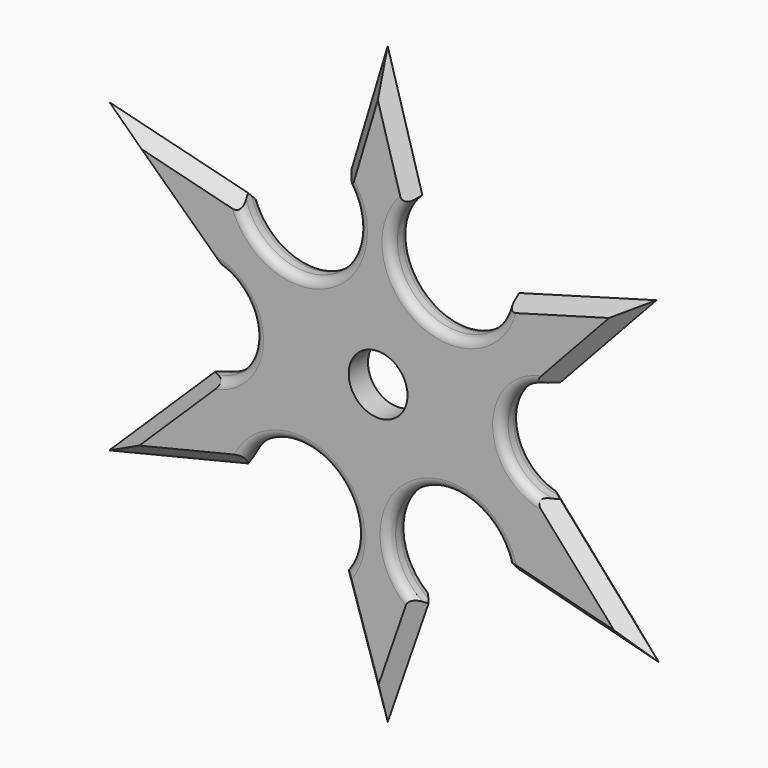
from build123d import *

# Parameters (mm, degrees)
F0_R         = 4.0240897433
F0_R_2       = 2.1702911965
F1_DEPTH     = 0.889
F2_DEPTH     = 0.889
F3_SIZE      = 1.016
F4_R         = 0.635
F5_T1_DEPTH  = 15.9932905978
F5_T3_DEPTH  = 16.1545129753
F5_T5_DEPTH  = 16.1936477888
F5_T7_DEPTH  = 16.3204160833
F5_T9_DEPTH  = 16.5038775979
F5_T11_DEPTH = 16.1754599615
F5_T13_DEPTH = 14.8813266149
F5_T15_DEPTH = 14.7778979971
F5_T17_DEPTH = 16.2458412717
F5_T19_DEPTH = 16.498961557
F5_T21_DEPTH = 14.852247235
F5_T23_DEPTH = 14.8224282878
F6_R         = 0.635


# Not quite as in the source:
# - a fillet or chamfer that OpenCascade refuses, or shapes differently, is made with other operations: its cross-section is extruded or revolved along the edge and cut away or added


with BuildPart() as f1:
    # F0 (on Front) → F1 (new body, symmetric)
    with BuildSketch(Plane.XZ):
        with BuildLine():
            ThreePointArc((-12.921775703, 3.9272087544), (-9.095056291, 0.1291059315), (-12.921775703, -3.6689968914))
            Line((-12.921775703, -3.6689968914), (-11.6317034987, -6.3241203273))
            Line((-11.6317034987, -6.3241203273), (-10.3416312944, -8.9792437632))
            ThreePointArc((-10.3416312944, -8.9792437632), (-3.7268534074, -6.4636823832), (-2.9634656604, -13.4993468649))
            Line((-2.9634656604, -13.4993468649), (0, -13.5794270365))
            Line((0, -13.5794270365), (3.1296215133, -13.6639971501))
            ThreePointArc((3.1296215133, -13.6639971501), (2.8041191173, -5.9768088987), (9.7185348855, -9.3516673562))
            Line((9.7185348855, -9.3516673562), (11.3201552942, -6.5125130277))
            Line((11.3201552942, -6.5125130277), (12.921775703, -3.6733586992))
            ThreePointArc((12.921775703, -3.6733586992), (9.0928589552, 0.1269250276), (12.921775703, 3.9272087544))
            Line((12.921775703, 3.9272087544), (11.3201552942, 6.4055448308))
            Line((11.3201552942, 6.4055448308), (9.7185348855, 8.8838809072))
            ThreePointArc((9.7185348855, 8.8838809072), (3.1603710023, 5.5177443003), (2.6637583381, 12.8725906642))
            Line((2.6637583381, 12.8725906642), (0, 12.8725906642))
            Line((0, 12.8725906642), (-2.7692650138, 12.8725906642))
            ThreePointArc((-2.7692650138, 12.8725906642), (-3.8215008101, 5.6879732844), (-10.3416312944, 8.8838809072))
            Line((-10.3416312944, 8.8838809072), (-11.6317034987, 6.4055448308))
            Line((-11.6317034987, 6.4055448308), (-12.921775703, 3.9272087544))
        make_face()
        Circle(F0_R, mode=Mode.SUBTRACT)
        Circle(F0_R)
        Circle(F0_R_2, mode=Mode.SUBTRACT)
    extrude(amount=F1_DEPTH, both=True)

    # F0 (on Front) → F2 (join, symmetric)
    with BuildSketch(Plane.XZ):
        Polygon((-16.3057108253, 8.9796162218), (-11.6317034987, 6.4055448308), (-10.3416312944, 8.8838809072), align=None)
        Polygon((-16.3057108253, 8.9796162218), (-12.921775703, 3.9272087544), (-11.6317034987, 6.4055448308), align=None)
        Polygon((-20.9797181518, 11.5536876128), (-12.921775703, 3.9272087544), (-16.3057108253, 8.9796162218), align=None)
        Polygon((-10.3416312944, 8.8838809072), (-20.9797181518, 11.5536876128), (-16.3057108253, 8.9796162218), align=None)
        Polygon((0, 17.4824267871), (-2.7692650138, 12.8725906642), (0, 12.8725906642), align=None)
        Polygon((0, 17.4824267871), (0, 12.8725906642), (2.6637583381, 12.8725906642), align=None)
        Polygon((2.6637583381, 12.8725906642), (0, 22.0922629099), (0, 17.4824267871), align=None)
        Polygon((0, 22.0922629099), (-2.7692650138, 12.8725906642), (0, 17.4824267871), align=None)
        Polygon((-16.378282755, -8.9792437632), (-20.9840265761, -11.5555872095), (-10.3416312944, -8.9792437632), align=None)
        Polygon((-16.378282755, -8.9792437632), (-12.921775703, -3.6689968914), (-20.9840265761, -11.5555872095), align=None)
        Polygon((-11.6317034987, -6.3241203273), (-12.921775703, -3.6689968914), (-16.378282755, -8.9792437632), align=None)
        Polygon((-10.3416312944, -8.9792437632), (-11.6317034987, -6.3241203273), (-16.378282755, -8.9792437632), align=None)
        Polygon((0, -18.7971512683), (-2.9634656604, -13.4993468649), (0, -22.6890025881), align=None)
        Polygon((0, -18.7971512683), (0, -22.6890025881), (3.1296215133, -13.6639971501), align=None)
        Polygon((3.1296215133, -13.6639971501), (0, -13.5794270365), (0, -18.7971512683), align=None)
        Polygon((0, -13.5794270365), (-2.9634656604, -13.4993468649), (0, -18.7971512683), align=None)
        Polygon((16.1898454279, -9.5265381722), (20.3846063865, -12.1228255452), (12.921775703, -3.6733586992), align=None)
        Polygon((12.921775703, -3.6733586992), (11.3201552942, -6.5125130277), (16.1898454279, -9.5265381722), align=None)
        Polygon((11.3201552942, -6.5125130277), (9.7185348855, -9.3516673562), (16.1898454279, -9.5265381722), align=None)
        Polygon((16.1898454279, -9.5265381722), (9.7185348855, -9.3516673562), (20.3846063865, -12.1228255452), align=None)
        Polygon((12.921775703, 3.9272087544), (20.2454214595, 11.8206291252), (15.7827883769, 9.113086978), align=None)
        Polygon((20.2454214595, 11.8206291252), (9.7185348855, 8.8838809072), (15.7827883769, 9.113086978), align=None)
        Polygon((15.7827883769, 9.113086978), (9.7185348855, 8.8838809072), (11.3201552942, 6.4055448308), align=None)
        Polygon((15.7827883769, 9.113086978), (11.3201552942, 6.4055448308), (12.921775703, 3.9272087544), align=None)
    extrude(amount=F2_DEPTH, both=True)

    # F3
    f3_edges = [f1.edges().sort_by_distance(p)[0] for p in [
        (-15.660675, -0.889, 10.218784),
        (-16.950747, -0.889, 7.740448),
        (-1.384633, -0.889, 17.482427),
        (1.331879, -0.889, 17.482427),
        (14.981978, -0.889, 10.352255),
        (16.583599, -0.889, 7.873919),
        (16.653191, -0.889, -7.898092),
        (15.051571, -0.889, -10.737246),
        (1.564811, -0.889, -18.1765),
        (-1.481733, -0.889, -18.094175),
        (-15.662829, -0.889, -10.267415),
        (-16.952901, -0.889, -7.612292),
    ]]
    chamfer(f3_edges, length=F3_SIZE)

    # F4
    f4_edges = [f1.edges().sort_by_distance(p)[0] for p in [
        (-3.69199, -0.889, -6.485261),
        (2.770724, -0.889, -5.998879),
        (9.093189, -0.889, 0.07683),
        (3.156805, -0.889, 5.519763),
        (-3.847037, -0.889, 5.674627),
        (-9.0961, -0.889, 0.040071),
    ]]
    fillet(f4_edges, radius=F4_R)

    # F5: chamfer of 1.016 on 12 edges, made by hand

    # F5_s2 → F5_t1 (cut)
    with BuildSketch(Plane(origin=(6.1587132778, 0, 6.6378569447), x_dir=(0, 1, 0), z_dir=(0.6801538719, 0, 0.7330693764))):
        Polygon((0.889, -5.7854518163), (-0.127, -6.8014518163), (0.889, -6.8014518163), align=None)
    extrude(amount=F5_T1_DEPTH, mode=Mode.SUBTRACT)

    # F5_s4 → F5_t3 (cut)
    with BuildSketch(Plane(origin=(24.3598265124, 0, 6.7958058252), x_dir=(0, 1, 0), z_dir=(-0.9632196934, 0, -0.2687151323))):
        Polygon((0.889, -4.9296116562), (-0.127, -5.9456116562), (0.889, -5.9456116562), align=None)
    extrude(amount=F5_T3_DEPTH, mode=Mode.SUBTRACT)

    # F5_s6 → F5_t5 (cut)
    with BuildSketch(Plane(origin=(-9.2920779296, 0, 2.3320031409), x_dir=(0, 1, 0), z_dir=(-0.9699214568, 0, 0.2434180924))):
        Polygon((-0.127, -6.0993265498), (0.889, -5.0833265498), (0.889, -6.0993265498), align=None)
    extrude(amount=F5_T5_DEPTH, mode=Mode.SUBTRACT)

    # F5_s8 → F5_t7 (cut)
    with BuildSketch(Plane(origin=(-18.7323182554, 0, 17.7292938056), x_dir=(0, 1, 0), z_dir=(0.7262838647, 0, -0.6873948995))):
        Polygon((0.889, -5.0140943587), (-0.127, -6.0300943587), (0.889, -6.0300943587), align=None)
    extrude(amount=F5_T7_DEPTH, mode=Mode.SUBTRACT)

    # F5_s10 → F5_t9 (cut)
    with BuildSketch(Plane(origin=(-6.5694590803, 0, -6.426323516), x_dir=(0, 1, 0), z_dir=(-0.7148514987, 0, -0.6992762936))):
        Polygon((0.889, -5.3971034937), (-0.127, -6.4131034937), (0.889, -6.4131034937), align=None)
    extrude(amount=F5_T9_DEPTH, mode=Mode.SUBTRACT)

    # F5_s12 → F5_t11 (cut)
    with BuildSketch(Plane(origin=(-25.0043780522, 0, -6.0531359546), x_dir=(0, 1, 0), z_dir=(0.9719259854, 0, 0.2352868012))):
        Polygon((0.889, -5.2779109968), (-0.127, -6.2939109968), (0.889, -6.2939109968), align=None)
    extrude(amount=F5_T11_DEPTH, mode=Mode.SUBTRACT)

    # F5_s14 → F5_t13 (cut)
    with BuildSketch(Plane(origin=(2.8621226494, 0, -8.8753928), x_dir=(0, 1, 0), z_dir=(0.3069146572, 0, -0.95173704))):
        Polygon((0.889, -5.9475874505), (-0.127, -6.9635874505), (0.889, -6.9635874505), align=None)
    extrude(amount=F5_T13_DEPTH, mode=Mode.SUBTRACT)

    # F5_s16 → F5_t15 (cut)
    with BuildSketch(Plane(origin=(-7.8793990178, 0, -22.7221146971), x_dir=(0, 1, 0), z_dir=(0.3276322741, 0, 0.9448053201))):
        Polygon((0.889, -6.4176495158), (-0.127, -7.4336495158), (0.889, -7.4336495158), align=None)
    extrude(amount=F5_T15_DEPTH, mode=Mode.SUBTRACT)

    # F5_s18 → F5_t17 (cut)
    with BuildSketch(Plane(origin=(8.8511554127, 0, -2.2996237933), x_dir=(0, 1, 0), z_dir=(0.9678671407, 0, -0.2514621201))):
        Polygon((0.889, -5.5913281585), (-0.127, -6.6073281585), (0.889, -6.6073281585), align=None)
    extrude(amount=F5_T17_DEPTH, mode=Mode.SUBTRACT)

    # F5_s20 → F5_t19 (cut)
    with BuildSketch(Plane(origin=(16.677859402, 0, -18.8827840339), x_dir=(0, 1, 0), z_dir=(-0.6619915678, 0, 0.7495112835))):
        Polygon((0.889, -6.2372842084), (-0.127, -7.2532842084), (0.889, -7.2532842084), align=None)
    extrude(amount=F5_T19_DEPTH, mode=Mode.SUBTRACT)

    # F5_s22 → F5_t21 (cut)
    with BuildSketch(Plane(origin=(6.8382387811, 0, 22.7664452427), x_dir=(0, 1, 0), z_dir=(-0.2876684019, 0, -0.9577300719))):
        Polygon((0.889, -5.3392459651), (-0.127, -6.3552459651), (0.889, -6.3552459651), align=None)
    extrude(amount=F5_T21_DEPTH, mode=Mode.SUBTRACT)

    # F5_s24 → F5_t23 (cut)
    with BuildSketch(Plane(origin=(-2.5021583411, 0, 8.6603501083), x_dir=(0, 1, 0), z_dir=(-0.2775682617, 0, 0.9607059176))):
        Polygon((0.889, -5.1161110124), (-0.127, -6.1321110124), (0.889, -6.1321110124), align=None)
    extrude(amount=F5_T23_DEPTH, mode=Mode.SUBTRACT)

    # F6
    f6_edges = [f1.edges().sort_by_distance(p)[0] for p in [
        (3.156805, 0.889, 5.519763),
        (-3.847037, 0.889, 5.674627),
        (-9.0961, 0.889, 0.040071),
        (-3.69199, 0.889, -6.485261),
        (2.770724, 0.889, -5.998879),
        (9.093189, 0.889, 0.07683),
    ]]
    fillet(f6_edges, radius=F6_R)


solid = f1.part
